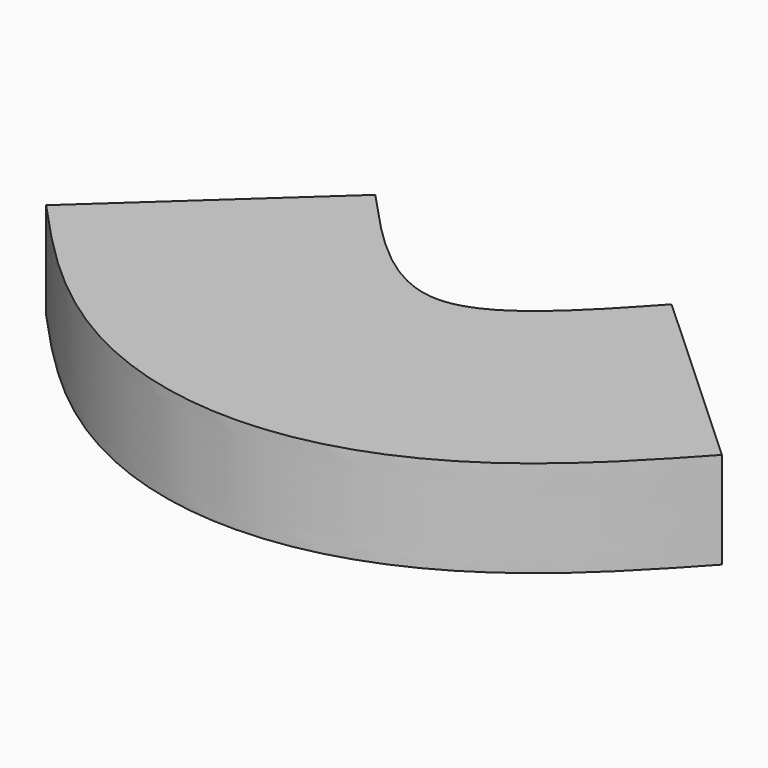
from build123d import *

# Parameters (mm, degrees)
F1_DEPTH = 19.05


# Not quite as in the source:
# - the dataset's text gives a spline's control points without its knots; the knots are read off the source's solid


with BuildPart() as f1:
    # F0 (on Top) → F1 (new body)
    with BuildSketch(Plane.XY):
        with BuildLine():
            add(Edge.make_bspline(
                [(-29.21, 50.1937808475), (-19.4733333333, 39.5917887583), (0, 18.38780458), (19.4733333333, 39.5917887583), (29.21, 50.1937808475)],
                knots=[0, 0, 0, 0, 0.5, 1, 1, 1, 1], degree=3))
            Line((-29.21, 50.1937808475), (-66.6254663511, 15.8321324917))
            add(Edge.make_bspline(
                [(-66.6254663511, 15.8321324917), (-65.4083830178, 14.5068834805), (-62.798118937, 11.6631929013), (-58.313838197, 6.9250114854), (-53.1264544051, 1.7899227882), (-48.0008550127, -2.7750884656), (-43.1855874656, -6.5540915551), (-39.1310205383, -9.4265922107), (-34.5338667026, -12.2947905426), (-29.2793634388, -15.0836296108), (-24.2551988213, -17.2389760424), (-19.805410967, -18.7668245668), (-16.2491616584, -19.783449029), (-12.4760888182, -20.637258157), (-9.1603044553, -21.1827909222), (-6.4154794436, -21.5013942758), (-4.3147237261, -21.677087596), (-2.5322491694, -21.7673504521), (-1.0905389143, -21.8040063692), (0, -21.8133018117), (1.0905389143, -21.8040063692), (2.5322491694, -21.7673504521), (4.3147237261, -21.677087596), (6.4154794436, -21.5013942758), (9.1603044553, -21.1827909222), (12.4760888182, -20.637258157), (16.2491616584, -19.783449029), (19.805410967, -18.7668245668), (24.2551988213, -17.2389760424), (29.2793634388, -15.0836296108), (34.5338667026, -12.2947905426), (39.1310205383, -9.4265922107), (43.1855874656, -6.5540915551), (48.0008550127, -2.7750884656), (53.1264544051, 1.7899227882), (58.313838197, 6.9250114854), (62.798118937, 11.6631929013), (65.4083830178, 14.5068834805), (66.6254663511, 15.8321324917)],
                knots=[0, 0, 0, 0, 0.0625, 0.125, 0.1875, 0.25, 0.28125, 0.3125, 0.34375, 0.375, 0.40625, 0.421875, 0.4375, 0.453125, 0.46875, 0.4765625, 0.484375, 0.4921875, 0.49609375, 0.5, 0.50390625, 0.5078125, 0.515625, 0.5234375, 0.53125, 0.546875, 0.5625, 0.578125, 0.59375, 0.625, 0.65625, 0.6875, 0.71875, 0.75, 0.8125, 0.875, 0.9375, 1, 1, 1, 1], degree=3))
            Line((66.6254663511, 15.8321324917), (29.21, 50.1937808475))
        make_face()
    extrude(amount=F1_DEPTH)


solid = f1.part
